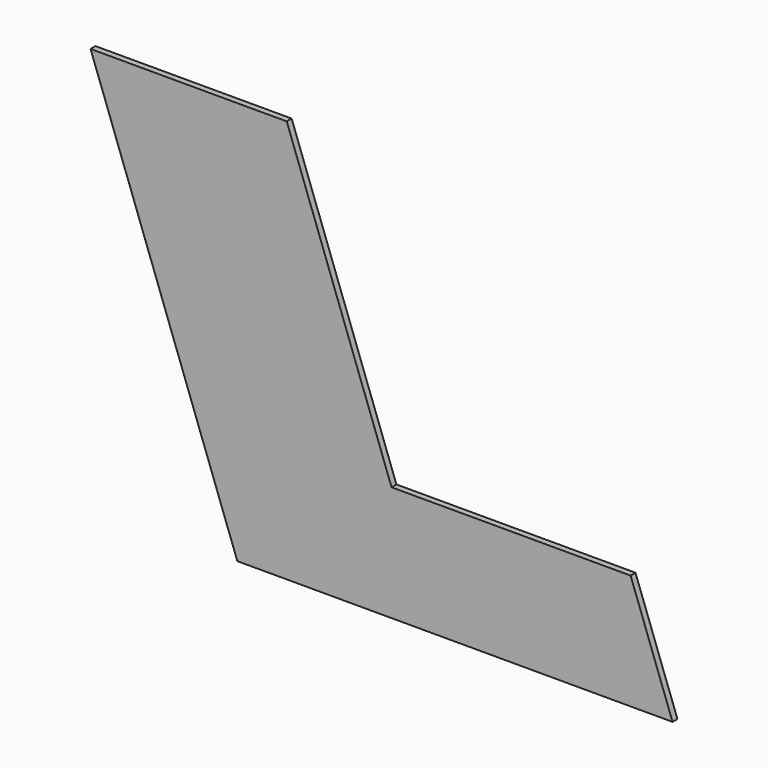
from build123d import *

# Parameters (mm, degrees)
F1_DEPTH = 10


# Not quite as in the source:
# - a feature names something its author has since deleted; it is built from what else it names


with BuildPart() as f1:
    # F0 (on Front) → F1 (new body)
    with BuildSketch(Plane.XZ):
        Polygon((-756.6513559012, 227.7144607794), (-517.2372555732, -430.0703737707), (192.7627444268, -430.0703737707), (124.3587157616, -242.1318496135), (-265.6412842384, -242.1318496135), (-436.6513559012, 227.7144607794), align=None)
    extrude(amount=F1_DEPTH)


solid = f1.part
